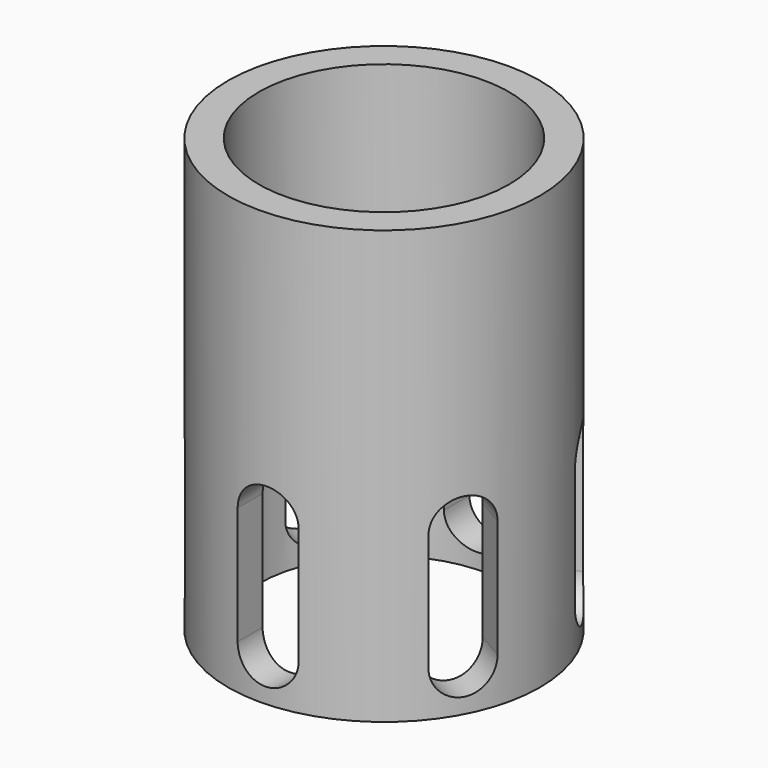
from build123d import *

# Parameters (mm, degrees)
F0_R            = 52.9622943823
F0_R_2          = 42.5146844638
F1_DEPTH        = 147
F3_REACH        = 97.6846539323
F3_COPIES_COUNT = 6


# Not quite as in the source:
# - a pattern or mirror of a feature is missing from the dataset's text; its kind, count and spacing are read off the source's solid


with BuildPart() as f1:
    # F0 (on Top) → F1 (new body)
    with BuildSketch(Plane.XY):
        with Locations((2.2072358988, 0)):
            Circle(F0_R)
        with Locations((2.2072358988, 0)):
            Circle(F0_R_2, mode=Mode.SUBTRACT)
    extrude(amount=F1_DEPTH)

    f3_end = f1.faces().sort_by_distance((-50.7550584835, 0, 73.5))[0]
    # F2 (on Front) → F3 (cut, up to a face of the model that its end follows)
    with BuildSketch(Plane.XZ):
        with BuildLine():
            ThreePointArc((10, 55.2122774348), (0, 45.2122774348), (-10, 55.2122774348))
            Line((-10, 55.2122774348), (-10, 15.2122774348))
            ThreePointArc((-10, 15.2122774348), (0, 25.2122774348), (10, 15.2122774348))
            Line((10, 15.2122774348), (10, 55.2122774348))
        make_face()
        with BuildLine():
            ThreePointArc((10, 15.2122774348), (0, 25.2122774348), (-10, 15.2122774348))
            Line((-10, 15.2122774348), (10, 15.2122774348))
        make_face()
        with BuildLine():
            Line((10, 55.2122774348), (-10, 55.2122774348))
            ThreePointArc((-10, 55.2122774348), (0, 45.2122774348), (10, 55.2122774348))
        make_face()
        with BuildLine():
            Line((10, 15.2122774348), (-10, 15.2122774348))
            ThreePointArc((-10, 15.2122774348), (0, 5.2122774348), (10, 15.2122774348))
        make_face()
        with BuildLine():
            ThreePointArc((10, 55.2122774348), (0, 65.2122774348), (-10, 55.2122774348))
            Line((-10, 55.2122774348), (10, 55.2122774348))
        make_face()
    f3_long = extrude(amount=-F3_REACH, mode=Mode.PRIVATE)
    f3 = split(f3_long, bisect_by=f3_end, keep=Keep.BOTTOM, mode=Mode.PRIVATE)
    add(f3, mode=Mode.SUBTRACT)

    # F3_copies: F3 ×6 about axis
    f3_copies_axis = Axis((2.207236, 0, 0), (0, 0, 1))
    for i in range(1, F3_COPIES_COUNT):
        add(f3.rotate(f3_copies_axis, i * 360 / F3_COPIES_COUNT), mode=Mode.SUBTRACT)


solid = f1.part
